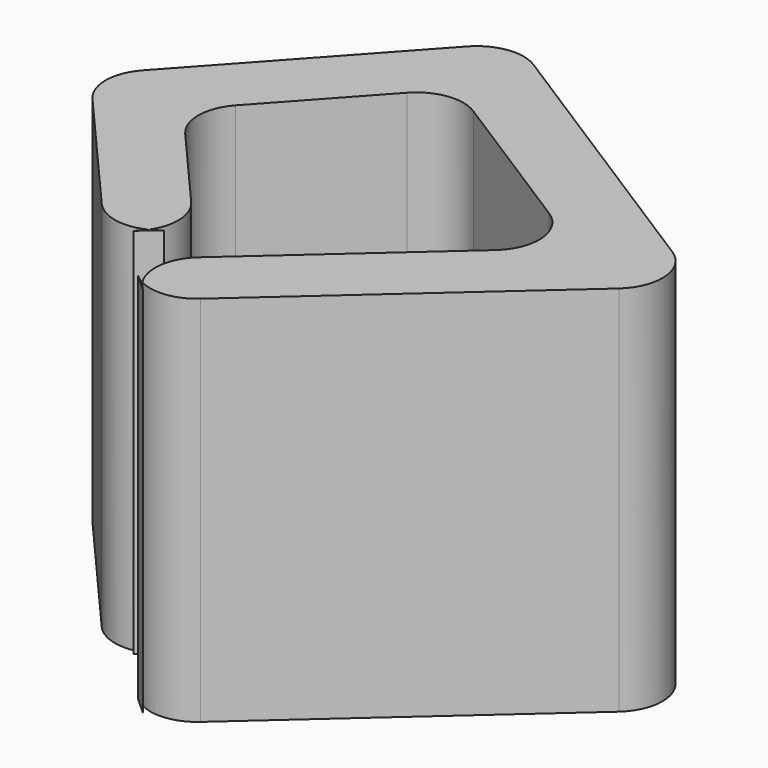
from build123d import *

# Parameters (mm, degrees)
F2_DEPTH = 444.5


# Not quite as in the source:
# - the program builds the solid bodies; features that only make, move or delete a surface that nothing else refers to are left out


with BuildPart() as f2:
    # F0 (on Top) → F2 (new body)
    with BuildSketch(Plane.XY):
        with BuildLine():
            ThreePointArc((27.9253781423, -261.9974371284), (22.9075756056, -256.8332185716), (18.5954934194, -251.0666387518))
            ThreePointArc((18.5954934194, -251.0666387518), (12.4265327198, -247.3529587055), (6.7863258601, -242.8768485437))
            Line((6.7863258601, -242.8768485437), (27.9253781423, -261.9974371284))
        make_face()
    extrude(amount=F2_DEPTH)


with BuildPart() as f2b:
    # F0 (on Top) → F2, piece 2 (new body)
    with BuildSketch(Plane.XY):
        with BuildLine():
            ThreePointArc((-31.1204911076, -156.4375346544), (-36.8123563953, -160.777560461), (-43.0123050994, -164.3544013187))
            ThreePointArc((-43.0123050994, -164.3544013187), (-47.417706923, -169.9958186255), (-52.5081003988, -175.0278210814))
            Line((-52.5081003988, -175.0278210814), (-31.1204911076, -156.4375346544))
        make_face()
    extrude(amount=F2_DEPTH)


with BuildPart() as f2c:
    # F0 (on Top) → F2, piece 3 (new body)
    with BuildSketch(Plane.XY):
        with BuildLine():
            Line((-248.9900153466, 9.0356711772), (-109.9539944558, -150.9214173747))
            ThreePointArc((-109.9539944558, -150.9214173747), (-78.773286297, -169.0505342784), (-43.0123050994, -164.3544013187))
            ThreePointArc((-43.0123050994, -164.3544013187), (-33.3817999447, -129.5958798966), (-46.991983119, -96.1943177332))
            Line((-46.991983119, -96.1943177332), (-137.3700341689, 7.7831251072))
            ThreePointArc((-137.3700341689, 7.7831251072), (-151.071705911, 45.068837312), (-136.5367849162, 82.0376919712))
            Line((-136.5367849162, 82.0376919712), (-27.7431442317, 201.6704729463))
            ThreePointArc((-27.7431442317, 201.6704729463), (6.1663489106, 219.4581595516), (43.5656902405, 211.2395959291))
            Line((43.5656902405, 211.2395959291), (227.7961883679, 94.1848714271))
            ThreePointArc((227.7961883679, 94.1848714271), (253.5267437249, 51.5283411547), (234.9918947151, 5.2887431239))
            Line((234.9918947151, 5.2887431239), (28.2474067267, -178.8241948134))
            ThreePointArc((28.2474067267, -178.8241948134), (10.0225407283, -213.1552626245), (18.5954934194, -251.0666387518))
            ThreePointArc((18.5954934194, -251.0666387518), (51.2422832265, -256.8782248907), (81.4343139607, -243.1658692103))
            Line((81.4343139607, -243.1658692103), (372.971118428, 16.4574857317))
            ThreePointArc((372.971118428, 16.4574857317), (391.5059674378, 62.6970837625), (365.7754120808, 105.3536140349))
            Line((365.7754120808, 105.3536140349), (29.0662717973, 319.2888530632))
            ThreePointArc((29.0662717973, 319.2888530632), (-8.3330695326, 327.5074166856), (-42.2425626749, 309.7197300804))
            Line((-42.2425626749, 309.7197300804), (-248.1567660939, 83.2902380412))
            ThreePointArc((-248.1567660939, 83.2902380412), (-262.6916870886, 46.3213833819), (-248.9900153466, 9.0356711772))
        make_face()
    extrude(amount=F2_DEPTH)


solid = Compound([f2.part, f2b.part, f2c.part])
